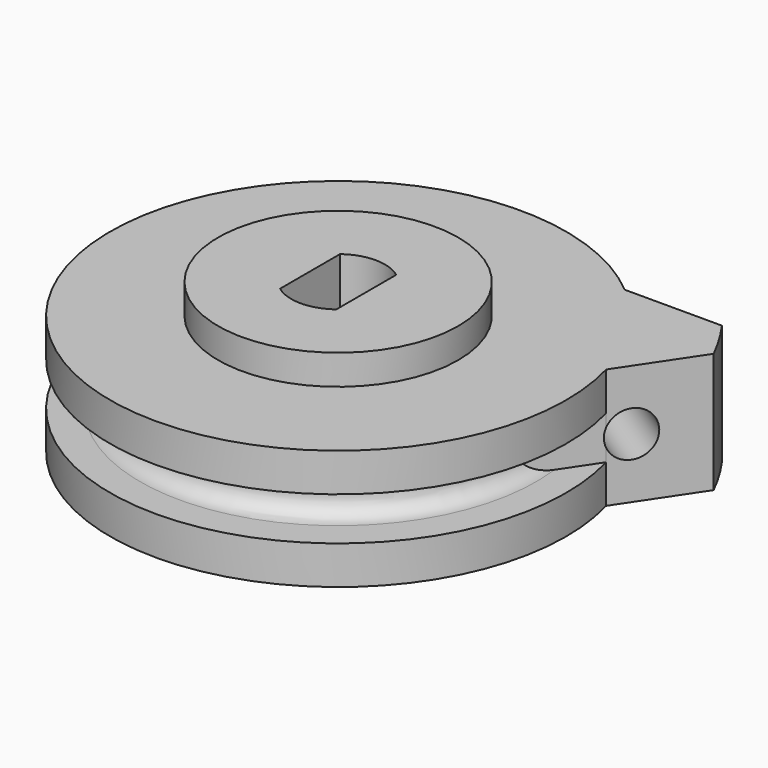
from build123d import *

# Parameters (mm, degrees)
F0_R          = 6.35
F1_DEPTH      = 1.5875
F2_R          = 9.525
F2_R_2        = 6.35
F3_DEPTH      = 6.35
F4_R          = 12.065
F4_R_2        = 9.525
F5_DEPTH      = 2.032
F6_R          = 12.065
F6_R_2        = 6.35
F7_DEPTH      = 2.032
F9_DEPTH      = 6.35
F10_R         = 1.2005117183
F11_DEPTH     = 12.7
F12_T1_DEPTH  = 3.6932202738
F12_T6_ANGLE  = 313.32464119
F12_S7_R      = 1.2005117183
F12_T8_DEPTH  = 18
F12_T12_DEPTH = 2.8797396175
F12_S13_R     = 1.2005117183
F12_T14_DEPTH = 3
F12_T18_ANGLE = 313.32464119
F12_S19_R     = 1.2005117183
F12_T20_DEPTH = 18


# Not quite as in the source:
# - a fillet or chamfer that OpenCascade refuses, or shapes differently, is made with other operations: its cross-section is extruded or revolved along the edge and cut away or added


with BuildPart() as f1:
    # F0 (on Top) → F1 (new body)
    with BuildSketch(Plane.XY):
        Circle(F0_R)
        with BuildLine():
            ThreePointArc((1.4859, -1.9812), (0, -2.4765), (-1.4859, -1.9812))
            Line((-1.4859, -1.9812), (-1.4859, 1.9812))
            ThreePointArc((-1.4859, 1.9812), (0, 2.4765), (1.4859, 1.9812))
            Line((1.4859, 1.9812), (1.4859, -1.9812))
        make_face(mode=Mode.SUBTRACT)
    extrude(amount=-F1_DEPTH)

    # F2 (on face) → F3 (join)
    with BuildSketch(Plane(origin=(0, 0, -1.5875), x_dir=(1, 0, 0), z_dir=(0, 0, -1))):
        Circle(F2_R)
        Circle(F2_R_2, mode=Mode.SUBTRACT)
        Circle(F2_R_2)
        with BuildLine():
            ThreePointArc((-1.4859, 1.9812), (0, 2.4765), (1.4859, 1.9812))
            Line((1.4859, 1.9812), (1.4859, -1.9812))
            ThreePointArc((1.4859, -1.9812), (0, -2.4765), (-1.4859, -1.9812))
            Line((-1.4859, -1.9812), (-1.4859, 1.9812))
        make_face(mode=Mode.SUBTRACT)
    extrude(amount=F3_DEPTH)

    # F4 (on face) → F5 (join)
    with BuildSketch(Plane.XY.offset(-1.5875)):
        Circle(F4_R)
        Circle(F4_R_2, mode=Mode.SUBTRACT)
    extrude(amount=-F5_DEPTH)

    # F6 (on face) → F7 (join)
    with BuildSketch(Plane(origin=(0, 0, -7.9375), x_dir=(1, 0, 0), z_dir=(0, 0, -1))):
        Circle(F6_R)
        Circle(F6_R_2, mode=Mode.SUBTRACT)
    extrude(amount=-F7_DEPTH)

    # F8 (on face) → F9 (join)
    with BuildSketch(Plane.XY.offset(-1.5875)):
        with BuildLine():
            ThreePointArc((7.7828940639, 9.2190446897), (10.1726283334, 6.4870530898), (11.6416666667, 3.1679365875))
            Line((11.6416666667, 3.1679365875), (14.2287037037, 7.0398590833))
            ThreePointArc((14.2287037037, 7.0398590833), (13.6199100402, 8.1555916706), (12.9238090364, 9.2190446897))
            Line((12.9238090364, 9.2190446897), (7.7828940639, 9.2190446897))
        make_face()
        with BuildLine():
            ThreePointArc((2.3947525988, 9.2190446897), (7.534442365, 5.8273324299), (9.525, 0))
            Line((9.525, 0), (11.6416666667, 3.1679365875))
            ThreePointArc((11.6416666667, 3.1679365875), (10.1726283334, 6.4870530898), (7.7828940639, 9.2190446897))
            Line((7.7828940639, 9.2190446897), (2.3947525988, 9.2190446897))
        make_face()
    extrude(amount=-F9_DEPTH)

    # F10 (on face) → F11 (cut)
    with BuildSketch(Plane(origin=(6.5851851852, -4.399911927, 0), x_dir=(0.5555555556, 0.8314794193, 0), z_dir=(0.8314794193, -0.5555555556, 0))):
        with Locations((10.2023333333, -4.7625)):
            Circle(F10_R)
    extrude(amount=-F11_DEPTH, mode=Mode.SUBTRACT)

    # F12: fillet of radius 0.9525 on 4 edges, made by hand

    # F12_s2 → F12_t1 (join)
    with BuildSketch(Plane.XY.offset(-6.6091101369)):
        with BuildLine():
            ThreePointArc((9.6813578082, 0.2340149392), (9.5658390102, -0.0058514421), (9.5212199592, -0.2683197522))
            ThreePointArc((9.5212199592, -0.2683197522), (9.5240549429, -0.1341731886), (9.525, 0))
            Line((9.525, 0), (9.6813578082, 0.2340149392))
        make_face()
    extrude(amount=F12_T1_DEPTH)


with BuildPart() as f12_tool4:
    # F12_s5 → F12_t6 (revolve)
    with BuildSketch(Plane(origin=(0, 0, 0), x_dir=(0, 0, 1), z_dir=(0.8751013478, -0.4839396977, 0))):
        with BuildLine():
            ThreePointArc((-3.6195, -10.4775), (-3.8984807909, -9.8039807909), (-4.572, -9.525))
            Line((-4.572, -9.525), (-3.6195, -9.525))
            Line((-3.6195, -9.525), (-3.6195, -10.4775))
        make_face()
    revolve(axis=Axis((0, 0, -3.6195), (0, 0, 1)), revolution_arc=F12_T6_ANGLE)

    # F12_s7 → F12_t8 (cut, symmetric)
    with BuildSketch(Plane(origin=(0, 0, 0), x_dir=(0, 0, 1), z_dir=(0.8314794193, -0.5555555556, 0))):
        with Locations((-4.7625, -10.2023333333)):
            Circle(F12_S7_R)
    extrude(amount=F12_T8_DEPTH, both=True, mode=Mode.SUBTRACT)


with BuildPart() as f1_1:
    add(f1.part)

    # F12_t3: union F12_tool4
    add(f12_tool4.part)


with BuildPart() as f12_tool10:
    # F12_s11 → F12_t12 (new body)
    with BuildSketch(Plane.XY.offset(-3.3226301913)):
        with BuildLine():
            ThreePointArc((2.2850004748, 9.2468588088), (2.398407194, 9.2260237879), (2.5135005223, 9.2190446897))
            Line((2.5135005223, 9.2190446897), (2.3947525988, 9.2190446897))
            ThreePointArc((2.3947525988, 9.2190446897), (2.3399178648, 9.2331148258), (2.2850004748, 9.2468588088))
        make_face()
    extrude(amount=-F12_T12_DEPTH)

    # F12_s13 → F12_t14 (cut, symmetric)
    with BuildSketch(Plane(origin=(-2.5775861998, 1.7222222222, 0), x_dir=(0, 0, 1), z_dir=(0.8314794193, -0.5555555556, 0))):
        with Locations((-4.7625, -10.2023333333)):
            Circle(F12_S13_R)
    extrude(amount=F12_T14_DEPTH, both=True, mode=Mode.SUBTRACT)


with BuildPart() as f1_2:
    add(f1_1.part)

    # F12_t9: union F12_tool10
    add(f12_tool10.part)


with BuildPart() as f12_tool16:
    # F12_s17 → F12_t18 (revolve)
    with BuildSketch(Plane(origin=(0, 0, 0), x_dir=(0, 0, 1), z_dir=(0.8751013478, -0.4839396977, 0))):
        with BuildLine():
            ThreePointArc((-5.9055, -10.4775), (-5.6265192091, -9.8039807909), (-4.953, -9.525))
            Line((-4.953, -9.525), (-5.9055, -9.525))
            Line((-5.9055, -9.525), (-5.9055, -10.4775))
        make_face()
    revolve(axis=Axis((0, 0, -5.9055), (0, 0, 1)), revolution_arc=F12_T18_ANGLE)

    # F12_s19 → F12_t20 (cut, symmetric)
    with BuildSketch(Plane(origin=(0, 0, 0), x_dir=(0, 0, 1), z_dir=(0.8314794193, -0.5555555556, 0))):
        with Locations((-4.7625, -10.2023333333)):
            Circle(F12_S19_R)
    extrude(amount=F12_T20_DEPTH, both=True, mode=Mode.SUBTRACT)


with BuildPart() as f1_3:
    add(f1_2.part)

    # F12_t15: union F12_tool16
    add(f12_tool16.part)


solid = f1_3.part
